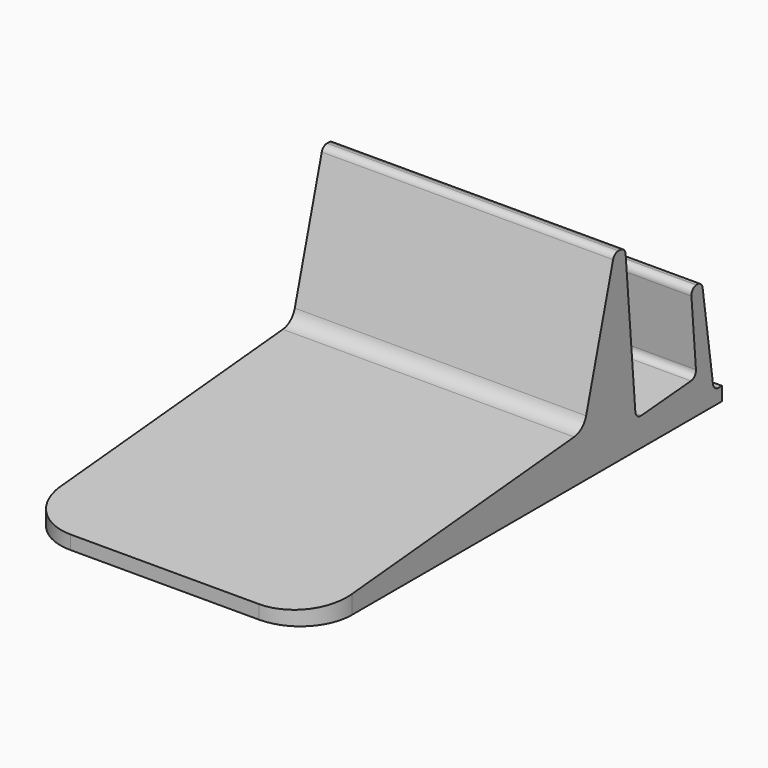
from build123d import *

# Parameters (mm, degrees)
F1_DEPTH = 85
F2_R     = 15
F3_R     = 2


# Not quite as in the source:
# - a feature of the source that left no trace in its solid (it failed there, or was rolled back) is left out


with BuildPart() as f1:
    # F0 (on Right) → F1 (new body)
    with BuildSketch(Plane.YZ):
        with BuildLine():
            Line((0, 4), (0, 0))
            Line((0, 0), (150, 0))
            Line((150, 0), (150, 4))
            Line((150, 4), (148.7324850447, 4))
            ThreePointArc((148.7324850447, 4), (147.4229901607, 4.4883045449), (146.7529275801, 5.7147768512))
            Line((146.7529275801, 5.7147768512), (142.6774710417, 34))
            Line((142.6774710417, 34), (138.7183561126, 33.4295537023))
            Line((138.7183561126, 33.4295537023), (140.5295339709, 11.9928994727))
            ThreePointArc((140.5295339709, 11.9928994727), (140.064889591, 10.5343894965), (138.7050141045, 9.8316203937))
            Line((138.7050141045, 9.8316203937), (120.5865966006, 8.3007995736))
            ThreePointArc((120.5865966006, 8.3007995736), (119.1280866244, 8.7654439535), (118.4253175217, 10.12531944))
            Line((118.4253175217, 10.12531944), (114.7183561126, 54))
            Line((114.7183561126, 54), (110.7183561126, 54))
            Line((110.7183561126, 54), (100.473891609, 16.4240136891))
            ThreePointArc((100.473891609, 16.4240136891), (98.862490978, 13.9077784109), (96.1038236872, 12.759820769))
            Line((96.1038236872, 12.759820769), (0, 4))
        make_face()
    extrude(amount=F1_DEPTH)

    # F2
    f2_edges = [f1.edges().sort_by_distance(p)[0] for p in [
        (85, 0, 2),
        (0, 0, 2),
    ]]
    fillet(f2_edges, radius=F2_R)

    # F3
    f3_edges = [f1.edges().sort_by_distance(p)[0] for p in [
        (42.5, 110.718356, 54),
        (42.5, 114.718356, 54),
        (42.5, 138.718356, 33.429554),
        (42.5, 142.677471, 34),
    ]]
    fillet(f3_edges, radius=F3_R)


solid = f1.part
